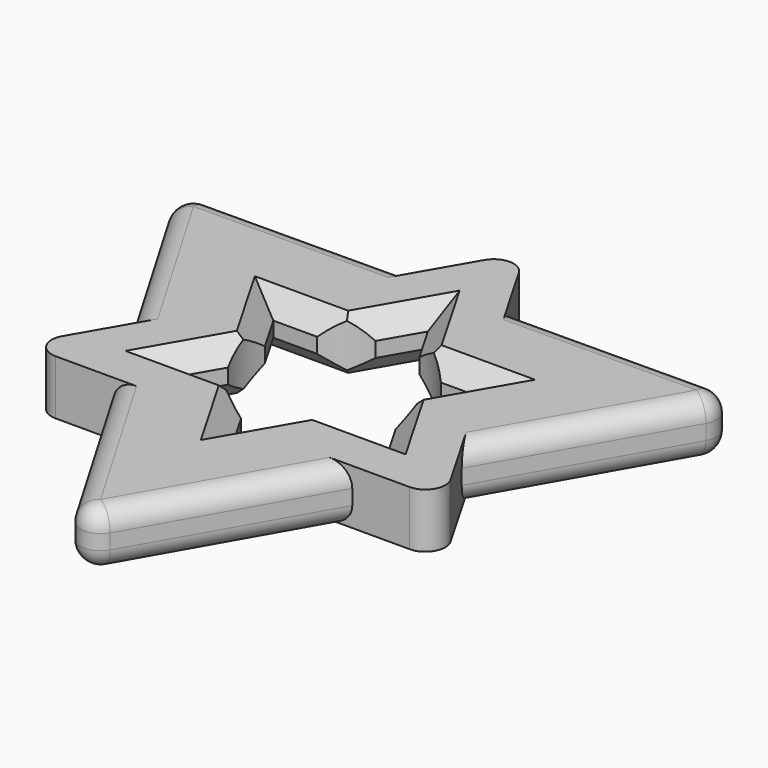
from build123d import *

# Parameters (mm, degrees)
F1_DEPTH      = 7
F2_T4_DEPTH   = 18.6684863764
F2_T9_DEPTH   = 18.6684863764
F2_T14_DEPTH  = 18.6684863764
F2_T19_DEPTH  = 18.6684863764
F2_T24_DEPTH  = 18.6684863764
F2_T29_DEPTH  = 18.6684863764
F2_T34_DEPTH  = 18.6684863764
F2_T39_DEPTH  = 18.6684863764
F2_T44_DEPTH  = 18.6684863764
F2_T49_DEPTH  = 18.6684863764
F2_T54_DEPTH  = 18.6684863764
F2_T59_DEPTH  = 18.6684863764
F2_T64_DEPTH  = 18.6684863764
F2_T69_DEPTH  = 18.6684863764
F2_T74_DEPTH  = 18.6684863764
F2_T79_DEPTH  = 18.6684863764
F2_T84_DEPTH  = 18.6684863764
F2_T89_DEPTH  = 18.6684863764
F2_T94_DEPTH  = 18.6684863764
F2_T99_DEPTH  = 18.6684863764
F2_T104_DEPTH = 18.6684863764
F2_T109_DEPTH = 18.6684863764
F2_T114_DEPTH = 18.6684863764
F2_T119_DEPTH = 18.6684863764
F2_T125_DEPTH = 18.6684863764
F2_T129_DEPTH = 18.6684863764
F2_T136_DEPTH = 18.6684863764
F2_T140_DEPTH = 18.6684863764
F2_T147_DEPTH = 18.6684863764
F2_T151_DEPTH = 18.6684863764
F2_T158_DEPTH = 18.6684863764
F2_T162_DEPTH = 18.6684863764
F2_T169_DEPTH = 18.6684863764
F2_T173_DEPTH = 18.6684863764
F2_T180_DEPTH = 18.6684863764
F2_T184_DEPTH = 18.6684863764
F2_T191_DEPTH = 18.6684863764
F2_T195_DEPTH = 18.6684863764
F2_T202_DEPTH = 18.6684863764
F2_T206_DEPTH = 18.6684863764
F2_T213_DEPTH = 18.6684863764
F2_T217_DEPTH = 18.6684863764
F2_T224_DEPTH = 18.6684863764
F2_T228_DEPTH = 18.6684863764
F2_T235_DEPTH = 18.6684863764
F2_T239_DEPTH = 18.6684863764
F2_T246_DEPTH = 18.6684863764
F2_T250_DEPTH = 18.6684863764
F3_R          = 2.54
F4_T1_DEPTH   = 28.9970452561
F4_T3_DEPTH   = 1.92
F4_T8_DEPTH   = 2.54
F4_T14_DEPTH  = 2.54
F4_T20_DEPTH  = 2.54
F4_T26_DEPTH  = 2.54
F4_T32_DEPTH  = 2.54
F4_T38_DEPTH  = 2.54


# Not quite as in the source:
# - a fillet or chamfer that OpenCascade refuses, or shapes differently, is made with other operations: its cross-section is extruded or revolved along the edge and cut away or added
# - two fillets or chamfers of one size are made in one step


with BuildPart() as f1:
    # F0 (on Top) → F1 (new body)
    with BuildSketch(Plane.XY):
        with BuildLine():
            Line((21.1293552338, -5.3833303027), (13.5159660258, 7.8034466234))
            ThreePointArc((13.5159660258, 7.8034466234), (15.0751012551, 4.0393612071), (15.6068932467, 0))
            ThreePointArc((15.6068932467, 0), (15.0751012551, -4.0393612071), (13.5159660258, -7.8034466234))
            ThreePointArc((13.5159660258, -7.8034466234), (7.8034466234, -13.5159660258), (0, -15.6068932467))
            Line((0, -15.6068932467), (15.3081617463, -15.6068932467))
            Line((15.3081617463, -15.6068932467), (21.1293552338, -5.3833303027))
        make_face()
        with BuildLine():
            ThreePointArc((0, 15.6068932467), (7.8034466234, 13.5159660258), (13.5159660258, 7.8034466234))
            Line((13.5159660258, 7.8034466234), (5.8618851526, 21.0607035809))
            Line((5.8618851526, 21.0607035809), (-5.9025768178, 20.9902235494))
            Line((-5.9025768178, 20.9902235494), (-13.5159660258, 7.8034466234))
            ThreePointArc((-13.5159660258, 7.8034466234), (-7.8034466234, 13.5159660258), (0, 15.6068932467))
        make_face()
        Polygon((5.8618851526, 21.0607035809), (13.5159660258, 7.8034466234), (21.1293552338, -5.3833303027), (36.2901170268, 21.2429968933), align=None)
        Polygon((-5.9025768178, 20.9902235494), (5.8618851526, 21.0607035809), (0, 31.2137864934), align=None)
        Polygon((27.0319320516, -15.6068932467), (21.1293552338, -5.3833303027), (15.3081617463, -15.6068932467), align=None)
        with BuildLine():
            Line((-15.226778416, -15.6068932467), (0, -15.6068932467))
            ThreePointArc((0, -15.6068932467), (-7.8034466234, -13.5159660258), (-13.5159660258, -7.8034466234))
            ThreePointArc((-13.5159660258, -7.8034466234), (-15.6068932467, 0), (-13.5159660258, 7.8034466234))
            Line((-13.5159660258, 7.8034466234), (-21.170046899, -5.4538103342))
            Line((-21.170046899, -5.4538103342), (-15.226778416, -15.6068932467))
        make_face()
        Polygon((15.3081617463, -15.6068932467), (0, -15.6068932467), (-15.226778416, -15.6068932467), (0.2519164487, -42.0496616981), align=None)
        Polygon((-21.170046899, -5.4538103342), (-13.5159660258, 7.8034466234), (-5.9025768178, 20.9902235494), (-36.5420334755, 20.8066648049), align=None)
        Polygon((-27.0319320516, -15.6068932467), (-15.226778416, -15.6068932467), (-21.170046899, -5.4538103342), align=None)
        with BuildLine():
            Line((-10.7137976271, 2.9499485854), (-13.5159660258, 7.8034466234))
            ThreePointArc((-13.5159660258, 7.8034466234), (-15.6068932467, 0), (-13.5159660258, -7.8034466234))
            Line((-13.5159660258, -7.8034466234), (-10.7137976271, -2.9499485854))
            ThreePointArc((-10.7137976271, -2.9499485854), (-11.1125, 0), (-10.7137976271, 2.9499485854))
        make_face()
        with BuildLine():
            ThreePointArc((2.8021683987, 10.7533952087), (5.55625, 9.6237072996), (7.9116292283, 7.8034466234))
            Line((7.9116292283, 7.8034466234), (13.5159660258, 7.8034466234))
            ThreePointArc((13.5159660258, 7.8034466234), (7.8034466234, 13.5159660258), (0, 15.6068932467))
            Line((0, 15.6068932467), (2.8021683987, 10.7533952087))
        make_face()
        with BuildLine():
            Line((13.5159660258, -7.8034466234), (7.9116292283, -7.8034466234))
            ThreePointArc((7.9116292283, -7.8034466234), (5.55625, -9.6237072996), (2.8021683987, -10.7533952087))
            Line((2.8021683987, -10.7533952087), (0, -15.6068932467))
            ThreePointArc((0, -15.6068932467), (7.8034466234, -13.5159660258), (13.5159660258, -7.8034466234))
        make_face()
        with BuildLine():
            ThreePointArc((-13.5159660258, -7.8034466234), (-7.8034466234, -13.5159660258), (0, -15.6068932467))
            Line((0, -15.6068932467), (-2.8021683987, -10.7533952087))
            ThreePointArc((-2.8021683987, -10.7533952087), (-5.55625, -9.6237072996), (-7.9116292283, -7.8034466234))
            Line((-7.9116292283, -7.8034466234), (-13.5159660258, -7.8034466234))
        make_face()
        with BuildLine():
            ThreePointArc((10.7137976271, 2.9499485854), (11.0123733223, 1.4883850509), (11.1125, 0))
            ThreePointArc((11.1125, 0), (11.0123733223, -1.4883850509), (10.7137976271, -2.9499485854))
            Line((10.7137976271, -2.9499485854), (13.5159660258, -7.8034466234))
            ThreePointArc((13.5159660258, -7.8034466234), (15.0751012551, -4.0393612071), (15.6068932467, 0))
            ThreePointArc((15.6068932467, 0), (15.0751012551, 4.0393612071), (13.5159660258, 7.8034466234))
            Line((13.5159660258, 7.8034466234), (10.7137976271, 2.9499485854))
        make_face()
        with BuildLine():
            Line((-2.8021683987, 10.7533952087), (0, 15.6068932467))
            ThreePointArc((0, 15.6068932467), (-7.8034466234, 13.5159660258), (-13.5159660258, 7.8034466234))
            Line((-13.5159660258, 7.8034466234), (-7.9116292283, 7.8034466234))
            ThreePointArc((-7.9116292283, 7.8034466234), (-5.55625, 9.6237072996), (-2.8021683987, 10.7533952087))
        make_face()
    extrude(amount=F1_DEPTH)

    # F2: chamfer of 2.54 on 24 edges, made by hand


with BuildPart() as f2_tool2:
    # F2_s3 → F2_t4 (new body)
    with BuildSketch(Plane.YZ.offset(-20.0480408152)):
        Polygon((7.8034466234, 4.46), (10.3434466234, 7), (7.8034466234, 7), align=None)
    extrude(amount=F2_T4_DEPTH)

    split(bisect_by=Plane(origin=(-6.7579830129, -3.9017233117, 0), x_dir=(0, 0, 1), z_dir=(0.8660254038, 0.5, 0)), keep=Keep.TOP)


with BuildPart() as f1_1:
    add(f1.part)

    # F2_t1: cut F2_tool2
    add(f2_tool2.part, mode=Mode.SUBTRACT)


with BuildPart() as f2_tool7:
    # F2_s8 → F2_t9 (new body)
    with BuildSketch(Plane.YZ.offset(-20.0480408152)):
        Polygon((7.8034466234, 2.54), (10.3434466234, 0), (7.8034466234, 0), align=None)
    extrude(amount=F2_T9_DEPTH)

    split(bisect_by=Plane(origin=(-6.7579830129, -3.9017233117, 0), x_dir=(0, 0, 1), z_dir=(0.8660254038, 0.5, 0)), keep=Keep.TOP)


with BuildPart() as f1_2:
    add(f1_1.part)

    # F2_t6: cut F2_tool7
    add(f2_tool7.part, mode=Mode.SUBTRACT)


with BuildPart() as f2_tool12:
    # F2_s13 → F2_t14 (new body)
    with BuildSketch(Plane(origin=(-0.6897772194, 1.19472919, 0), x_dir=(0, 0, 1), z_dir=(-0.5, 0.8660254038, 0))):
        Polygon((2.54, -7.8034466234), (0, -10.3434466234), (0, -7.8034466234), align=None)
    extrude(amount=F2_T14_DEPTH)

    split(bisect_by=Plane.XZ.offset(-7.8034466234), keep=Keep.TOP)


with BuildPart() as f1_3:
    add(f1_2.part)

    # F2_t11: cut F2_tool12
    add(f2_tool12.part, mode=Mode.SUBTRACT)


with BuildPart() as f2_tool17:
    # F2_s18 → F2_t19 (new body)
    with BuildSketch(Plane.YZ.offset(-1.3795544389)):
        Polygon((-7.8034466234, 2.54), (-10.3434466234, 0), (-7.8034466234, 0), align=None)
    extrude(amount=-F2_T19_DEPTH)

    split(bisect_by=Plane(origin=(-6.7579830129, 3.9017233117, 0), x_dir=(0, 0, 1), z_dir=(0.8660254038, -0.5, 0)), keep=Keep.TOP)


with BuildPart() as f1_4:
    add(f1_3.part)

    # F2_t16: cut F2_tool17
    add(f2_tool17.part, mode=Mode.SUBTRACT)


with BuildPart() as f2_tool22:
    # F2_s23 → F2_t24 (new body)
    with BuildSketch(Plane(origin=(-10.0240204076, -17.3621126421, 0), x_dir=(0, 0, 1), z_dir=(0.5, 0.8660254038, 0))):
        Polygon((2.54, -7.8034466234), (0, -10.3434466234), (0, -7.8034466234), align=None)
    extrude(amount=F2_T24_DEPTH)

    split(bisect_by=Plane.XZ.offset(7.8034466234), keep=Keep.BOTTOM)


with BuildPart() as f1_5:
    add(f1_4.part)

    # F2_t21: cut F2_tool22
    add(f2_tool22.part, mode=Mode.SUBTRACT)


with BuildPart() as f2_tool27:
    # F2_s28 → F2_t29 (new body)
    with BuildSketch(Plane(origin=(10.0240204076, -17.3621126421, 0), x_dir=(0, 0, 1), z_dir=(-0.5, 0.8660254038, 0))):
        Polygon((2.54, -7.8034466234), (0, -10.3434466234), (0, -7.8034466234), align=None)
    extrude(amount=F2_T29_DEPTH)

    split(bisect_by=Plane(origin=(6.7579830129, -3.9017233117, 0), x_dir=(0, 0, 1), z_dir=(-0.8660254038, 0.5, 0)), keep=Keep.TOP)


with BuildPart() as f1_6:
    add(f1_5.part)

    # F2_t26: cut F2_tool27
    add(f2_tool27.part, mode=Mode.SUBTRACT)


with BuildPart() as f2_tool32:
    # F2_s33 → F2_t34 (new body)
    with BuildSketch(Plane(origin=(-0.6897772194, -1.19472919, 0), x_dir=(0, 0, 1), z_dir=(-0.5, -0.8660254038, 0))):
        Polygon((2.54, -7.8034466234), (0, -10.3434466234), (0, -7.8034466234), align=None)
    extrude(amount=F2_T34_DEPTH)

    split(bisect_by=Plane(origin=(-6.7579830129, -3.9017233117, 0), x_dir=(0, 0, 1), z_dir=(0.8660254038, 0.5, 0)), keep=Keep.TOP)


with BuildPart() as f1_7:
    add(f1_6.part)

    # F2_t31: cut F2_tool32
    add(f2_tool32.part, mode=Mode.SUBTRACT)


with BuildPart() as f2_tool37:
    # F2_s38 → F2_t39 (new body)
    with BuildSketch(Plane.YZ.offset(20.0480408152)):
        Polygon((-7.8034466234, 2.54), (-10.3434466234, 0), (-7.8034466234, 0), align=None)
    extrude(amount=-F2_T39_DEPTH)

    split(bisect_by=Plane(origin=(6.7579830129, 3.9017233117, 0), x_dir=(0, 0, 1), z_dir=(-0.8660254038, -0.5, 0)), keep=Keep.TOP)


with BuildPart() as f1_8:
    add(f1_7.part)

    # F2_t36: cut F2_tool37
    add(f2_tool37.part, mode=Mode.SUBTRACT)


with BuildPart() as f2_tool42:
    # F2_s43 → F2_t44 (new body)
    with BuildSketch(Plane(origin=(0.6897772194, -1.19472919, 0), x_dir=(0, 0, 1), z_dir=(0.5, -0.8660254038, 0))):
        Polygon((2.54, -7.8034466234), (0, -10.3434466234), (0, -7.8034466234), align=None)
    extrude(amount=F2_T44_DEPTH)

    split(bisect_by=Plane.XZ.offset(7.8034466234), keep=Keep.BOTTOM)


with BuildPart() as f1_9:
    add(f1_8.part)

    # F2_t41: cut F2_tool42
    add(f2_tool42.part, mode=Mode.SUBTRACT)


with BuildPart() as f2_tool47:
    # F2_s48 → F2_t49 (new body)
    with BuildSketch(Plane(origin=(10.0240204076, 17.3621126421, 0), x_dir=(0, 0, 1), z_dir=(-0.5, -0.8660254038, 0))):
        Polygon((2.54, -7.8034466234), (0, -10.3434466234), (0, -7.8034466234), align=None)
    extrude(amount=F2_T49_DEPTH)

    split(bisect_by=Plane.XZ.offset(-7.8034466234), keep=Keep.TOP)


with BuildPart() as f1_10:
    add(f1_9.part)

    # F2_t46: cut F2_tool47
    add(f2_tool47.part, mode=Mode.SUBTRACT)


with BuildPart() as f2_tool52:
    # F2_s53 → F2_t54 (new body)
    with BuildSketch(Plane.YZ.offset(1.3795544389)):
        Polygon((7.8034466234, 2.54), (10.3434466234, 0), (7.8034466234, 0), align=None)
    extrude(amount=F2_T54_DEPTH)

    split(bisect_by=Plane(origin=(6.7579830129, -3.9017233117, 0), x_dir=(0, 0, 1), z_dir=(-0.8660254038, 0.5, 0)), keep=Keep.TOP)


with BuildPart() as f1_11:
    add(f1_10.part)

    # F2_t51: cut F2_tool52
    add(f2_tool52.part, mode=Mode.SUBTRACT)


with BuildPart() as f2_tool57:
    # F2_s58 → F2_t59 (new body)
    with BuildSketch(Plane(origin=(-10.0240204076, 17.3621126421, 0), x_dir=(0, 0, 1), z_dir=(0.5, -0.8660254038, 0))):
        Polygon((2.54, -7.8034466234), (0, -10.3434466234), (0, -7.8034466234), align=None)
    extrude(amount=F2_T59_DEPTH)

    split(bisect_by=Plane(origin=(-6.7579830129, 3.9017233117, 0), x_dir=(0, 0, 1), z_dir=(0.8660254038, -0.5, 0)), keep=Keep.TOP)


with BuildPart() as f1_12:
    add(f1_11.part)

    # F2_t56: cut F2_tool57
    add(f2_tool57.part, mode=Mode.SUBTRACT)


with BuildPart() as f2_tool62:
    # F2_s63 → F2_t64 (new body)
    with BuildSketch(Plane(origin=(0.6897772194, 1.19472919, 0), x_dir=(0, 0, 1), z_dir=(0.5, 0.8660254038, 0))):
        Polygon((2.54, -7.8034466234), (0, -10.3434466234), (0, -7.8034466234), align=None)
    extrude(amount=F2_T64_DEPTH)

    split(bisect_by=Plane(origin=(6.7579830129, 3.9017233117, 0), x_dir=(0, 0, 1), z_dir=(-0.8660254038, -0.5, 0)), keep=Keep.TOP)


with BuildPart() as f1_13:
    add(f1_12.part)

    # F2_t61: cut F2_tool62
    add(f2_tool62.part, mode=Mode.SUBTRACT)


with BuildPart() as f2_tool67:
    # F2_s68 → F2_t69 (new body)
    with BuildSketch(Plane(origin=(0.6897772194, 1.19472919, 0), x_dir=(0, 0, 1), z_dir=(0.5, 0.8660254038, 0))):
        Polygon((4.46, -7.8034466234), (7, -10.3434466234), (7, -7.8034466234), align=None)
    extrude(amount=F2_T69_DEPTH)

    split(bisect_by=Plane(origin=(6.7579830129, 3.9017233117, 0), x_dir=(0, 0, 1), z_dir=(-0.8660254038, -0.5, 0)), keep=Keep.TOP)


with BuildPart() as f1_14:
    add(f1_13.part)

    # F2_t66: cut F2_tool67
    add(f2_tool67.part, mode=Mode.SUBTRACT)


with BuildPart() as f2_tool72:
    # F2_s73 → F2_t74 (new body)
    with BuildSketch(Plane(origin=(-10.0240204076, 17.3621126421, 0), x_dir=(0, 0, 1), z_dir=(0.5, -0.8660254038, 0))):
        Polygon((4.46, -7.8034466234), (7, -10.3434466234), (7, -7.8034466234), align=None)
    extrude(amount=F2_T74_DEPTH)

    split(bisect_by=Plane(origin=(-6.7579830129, 3.9017233117, 0), x_dir=(0, 0, 1), z_dir=(0.8660254038, -0.5, 0)), keep=Keep.TOP)


with BuildPart() as f1_15:
    add(f1_14.part)

    # F2_t71: cut F2_tool72
    add(f2_tool72.part, mode=Mode.SUBTRACT)


with BuildPart() as f2_tool77:
    # F2_s78 → F2_t79 (new body)
    with BuildSketch(Plane.YZ.offset(1.3795544389)):
        Polygon((7.8034466234, 4.46), (10.3434466234, 7), (7.8034466234, 7), align=None)
    extrude(amount=F2_T79_DEPTH)

    split(bisect_by=Plane(origin=(6.7579830129, -3.9017233117, 0), x_dir=(0, 0, 1), z_dir=(-0.8660254038, 0.5, 0)), keep=Keep.TOP)


with BuildPart() as f1_16:
    add(f1_15.part)

    # F2_t76: cut F2_tool77
    add(f2_tool77.part, mode=Mode.SUBTRACT)


with BuildPart() as f2_tool82:
    # F2_s83 → F2_t84 (new body)
    with BuildSketch(Plane(origin=(10.0240204076, 17.3621126421, 0), x_dir=(0, 0, 1), z_dir=(-0.5, -0.8660254038, 0))):
        Polygon((4.46, -7.8034466234), (7, -10.3434466234), (7, -7.8034466234), align=None)
    extrude(amount=F2_T84_DEPTH)

    split(bisect_by=Plane.XZ.offset(-7.8034466234), keep=Keep.TOP)


with BuildPart() as f1_17:
    add(f1_16.part)

    # F2_t81: cut F2_tool82
    add(f2_tool82.part, mode=Mode.SUBTRACT)


with BuildPart() as f2_tool87:
    # F2_s88 → F2_t89 (new body)
    with BuildSketch(Plane(origin=(0.6897772194, -1.19472919, 0), x_dir=(0, 0, 1), z_dir=(0.5, -0.8660254038, 0))):
        Polygon((4.46, -7.8034466234), (7, -10.3434466234), (7, -7.8034466234), align=None)
    extrude(amount=F2_T89_DEPTH)

    split(bisect_by=Plane.XZ.offset(7.8034466234), keep=Keep.BOTTOM)


with BuildPart() as f1_18:
    add(f1_17.part)

    # F2_t86: cut F2_tool87
    add(f2_tool87.part, mode=Mode.SUBTRACT)


with BuildPart() as f2_tool92:
    # F2_s93 → F2_t94 (new body)
    with BuildSketch(Plane.YZ.offset(20.0480408152)):
        Polygon((-7.8034466234, 4.46), (-10.3434466234, 7), (-7.8034466234, 7), align=None)
    extrude(amount=-F2_T94_DEPTH)

    split(bisect_by=Plane(origin=(6.7579830129, 3.9017233117, 0), x_dir=(0, 0, 1), z_dir=(-0.8660254038, -0.5, 0)), keep=Keep.TOP)


with BuildPart() as f1_19:
    add(f1_18.part)

    # F2_t91: cut F2_tool92
    add(f2_tool92.part, mode=Mode.SUBTRACT)


with BuildPart() as f2_tool97:
    # F2_s98 → F2_t99 (new body)
    with BuildSketch(Plane(origin=(-0.6897772194, -1.19472919, 0), x_dir=(0, 0, 1), z_dir=(-0.5, -0.8660254038, 0))):
        Polygon((4.46, -7.8034466234), (7, -10.3434466234), (7, -7.8034466234), align=None)
    extrude(amount=F2_T99_DEPTH)

    split(bisect_by=Plane(origin=(-6.7579830129, -3.9017233117, 0), x_dir=(0, 0, 1), z_dir=(0.8660254038, 0.5, 0)), keep=Keep.TOP)


with BuildPart() as f1_20:
    add(f1_19.part)

    # F2_t96: cut F2_tool97
    add(f2_tool97.part, mode=Mode.SUBTRACT)


with BuildPart() as f2_tool102:
    # F2_s103 → F2_t104 (new body)
    with BuildSketch(Plane(origin=(10.0240204076, -17.3621126421, 0), x_dir=(0, 0, 1), z_dir=(-0.5, 0.8660254038, 0))):
        Polygon((4.46, -7.8034466234), (7, -10.3434466234), (7, -7.8034466234), align=None)
    extrude(amount=F2_T104_DEPTH)

    split(bisect_by=Plane(origin=(6.7579830129, -3.9017233117, 0), x_dir=(0, 0, 1), z_dir=(-0.8660254038, 0.5, 0)), keep=Keep.TOP)


with BuildPart() as f1_21:
    add(f1_20.part)

    # F2_t101: cut F2_tool102
    add(f2_tool102.part, mode=Mode.SUBTRACT)


with BuildPart() as f2_tool107:
    # F2_s108 → F2_t109 (new body)
    with BuildSketch(Plane.YZ.offset(-1.3795544389)):
        Polygon((-7.8034466234, 4.46), (-10.3434466234, 7), (-7.8034466234, 7), align=None)
    extrude(amount=-F2_T109_DEPTH)

    split(bisect_by=Plane(origin=(-6.7579830129, 3.9017233117, 0), x_dir=(0, 0, 1), z_dir=(0.8660254038, -0.5, 0)), keep=Keep.TOP)


with BuildPart() as f1_22:
    add(f1_21.part)

    # F2_t106: cut F2_tool107
    add(f2_tool107.part, mode=Mode.SUBTRACT)


with BuildPart() as f2_tool112:
    # F2_s113 → F2_t114 (new body)
    with BuildSketch(Plane(origin=(-10.0240204076, -17.3621126421, 0), x_dir=(0, 0, 1), z_dir=(0.5, 0.8660254038, 0))):
        Polygon((4.46, -7.8034466234), (7, -10.3434466234), (7, -7.8034466234), align=None)
    extrude(amount=F2_T114_DEPTH)

    split(bisect_by=Plane.XZ.offset(7.8034466234), keep=Keep.BOTTOM)


with BuildPart() as f1_23:
    add(f1_22.part)

    # F2_t111: cut F2_tool112
    add(f2_tool112.part, mode=Mode.SUBTRACT)


with BuildPart() as f2_tool117:
    # F2_s118 → F2_t119 (new body)
    with BuildSketch(Plane(origin=(-0.6897772194, 1.19472919, 0), x_dir=(0, 0, 1), z_dir=(-0.5, 0.8660254038, 0))):
        Polygon((4.46, -7.8034466234), (7, -10.3434466234), (7, -7.8034466234), align=None)
    extrude(amount=F2_T119_DEPTH)

    split(bisect_by=Plane.XZ.offset(-7.8034466234), keep=Keep.TOP)


with BuildPart() as f1_24:
    add(f1_23.part)

    # F2_t116: cut F2_tool117
    add(f2_tool117.part, mode=Mode.SUBTRACT)


with BuildPart() as f2_tool123:
    # F2_s124 → F2_t125 (new body)
    with BuildSketch(Plane(origin=(-0.6897772194, 1.19472919, 0), x_dir=(0, 0, 1), z_dir=(-0.5, 0.8660254038, 0))):
        Polygon((4.46, -7.8034466234), (7, -10.3434466234), (7, -7.8034466234), align=None)
    extrude(amount=F2_T125_DEPTH)

    split(bisect_by=Plane.XZ.offset(-7.8034466234), keep=Keep.BOTTOM)


with BuildPart() as f2_tool127:
    # F2_s128 → F2_t129 (new body)
    with BuildSketch(Plane.YZ.offset(-20.0480408152)):
        Polygon((7.8034466234, 4.46), (10.3434466234, 7), (7.8034466234, 7), align=None)
    extrude(amount=F2_T129_DEPTH)

    split(bisect_by=Plane(origin=(-6.7579830129, -3.9017233117, 0), x_dir=(0, 0, 1), z_dir=(-0.8660254038, -0.5, 0)), keep=Keep.TOP)


with BuildPart() as f2_tool123_1:
    add(f2_tool123.part)

    # F2_t131: intersect F2_tool127
    add(f2_tool127.part, mode=Mode.INTERSECT)


with BuildPart() as f1_25:
    add(f1_24.part)

    # F2_t121: cut F2_tool123
    add(f2_tool123_1.part, mode=Mode.SUBTRACT)


with BuildPart() as f2_tool134:
    # F2_s135 → F2_t136 (new body)
    with BuildSketch(Plane(origin=(-0.6897772194, 1.19472919, 0), x_dir=(0, 0, 1), z_dir=(-0.5, 0.8660254038, 0))):
        Polygon((2.54, -7.8034466234), (0, -10.3434466234), (0, -7.8034466234), align=None)
    extrude(amount=F2_T136_DEPTH)

    split(bisect_by=Plane.XZ.offset(-7.8034466234), keep=Keep.BOTTOM)


with BuildPart() as f2_tool138:
    # F2_s139 → F2_t140 (new body)
    with BuildSketch(Plane.YZ.offset(-20.0480408152)):
        Polygon((7.8034466234, 2.54), (10.3434466234, 0), (7.8034466234, 0), align=None)
    extrude(amount=F2_T140_DEPTH)

    split(bisect_by=Plane(origin=(-6.7579830129, -3.9017233117, 0), x_dir=(0, 0, 1), z_dir=(-0.8660254038, -0.5, 0)), keep=Keep.TOP)


with BuildPart() as f2_tool134_1:
    add(f2_tool134.part)

    # F2_t142: intersect F2_tool138
    add(f2_tool138.part, mode=Mode.INTERSECT)


with BuildPart() as f1_26:
    add(f1_25.part)

    # F2_t132: cut F2_tool134
    add(f2_tool134_1.part, mode=Mode.SUBTRACT)


with BuildPart() as f2_tool145:
    # F2_s146 → F2_t147 (new body)
    with BuildSketch(Plane.YZ.offset(-1.3795544389)):
        Polygon((-7.8034466234, 2.54), (-10.3434466234, 0), (-7.8034466234, 0), align=None)
    extrude(amount=-F2_T147_DEPTH)

    split(bisect_by=Plane(origin=(-6.7579830129, 3.9017233117, 0), x_dir=(0, 0, 1), z_dir=(-0.8660254038, 0.5, 0)), keep=Keep.TOP)


with BuildPart() as f2_tool149:
    # F2_s150 → F2_t151 (new body)
    with BuildSketch(Plane(origin=(-10.0240204076, -17.3621126421, 0), x_dir=(0, 0, 1), z_dir=(0.5, 0.8660254038, 0))):
        Polygon((2.54, -7.8034466234), (0, -10.3434466234), (0, -7.8034466234), align=None)
    extrude(amount=F2_T151_DEPTH)

    split(bisect_by=Plane.XZ.offset(7.8034466234), keep=Keep.TOP)


with BuildPart() as f2_tool145_1:
    add(f2_tool145.part)

    # F2_t153: intersect F2_tool149
    add(f2_tool149.part, mode=Mode.INTERSECT)


with BuildPart() as f1_27:
    add(f1_26.part)

    # F2_t143: cut F2_tool145
    add(f2_tool145_1.part, mode=Mode.SUBTRACT)


with BuildPart() as f2_tool156:
    # F2_s157 → F2_t158 (new body)
    with BuildSketch(Plane(origin=(-0.6897772194, -1.19472919, 0), x_dir=(0, 0, 1), z_dir=(-0.5, -0.8660254038, 0))):
        Polygon((2.54, -7.8034466234), (0, -10.3434466234), (0, -7.8034466234), align=None)
    extrude(amount=F2_T158_DEPTH)

    split(bisect_by=Plane(origin=(-6.7579830129, -3.9017233117, 0), x_dir=(0, 0, 1), z_dir=(-0.8660254038, -0.5, 0)), keep=Keep.TOP)


with BuildPart() as f2_tool160:
    # F2_s161 → F2_t162 (new body)
    with BuildSketch(Plane(origin=(10.0240204076, -17.3621126421, 0), x_dir=(0, 0, 1), z_dir=(-0.5, 0.8660254038, 0))):
        Polygon((2.54, -7.8034466234), (0, -10.3434466234), (0, -7.8034466234), align=None)
    extrude(amount=F2_T162_DEPTH)

    split(bisect_by=Plane(origin=(6.7579830129, -3.9017233117, 0), x_dir=(0, 0, 1), z_dir=(0.8660254038, -0.5, 0)), keep=Keep.TOP)


with BuildPart() as f2_tool156_1:
    add(f2_tool156.part)

    # F2_t164: intersect F2_tool160
    add(f2_tool160.part, mode=Mode.INTERSECT)


with BuildPart() as f1_28:
    add(f1_27.part)

    # F2_t154: cut F2_tool156
    add(f2_tool156_1.part, mode=Mode.SUBTRACT)


with BuildPart() as f2_tool167:
    # F2_s168 → F2_t169 (new body)
    with BuildSketch(Plane(origin=(0.6897772194, -1.19472919, 0), x_dir=(0, 0, 1), z_dir=(0.5, -0.8660254038, 0))):
        Polygon((2.54, -7.8034466234), (0, -10.3434466234), (0, -7.8034466234), align=None)
    extrude(amount=F2_T169_DEPTH)

    split(bisect_by=Plane.XZ.offset(7.8034466234), keep=Keep.TOP)


with BuildPart() as f2_tool171:
    # F2_s172 → F2_t173 (new body)
    with BuildSketch(Plane.YZ.offset(20.0480408152)):
        Polygon((-7.8034466234, 2.54), (-10.3434466234, 0), (-7.8034466234, 0), align=None)
    extrude(amount=-F2_T173_DEPTH)

    split(bisect_by=Plane(origin=(6.7579830129, 3.9017233117, 0), x_dir=(0, 0, 1), z_dir=(0.8660254038, 0.5, 0)), keep=Keep.TOP)


with BuildPart() as f2_tool167_1:
    add(f2_tool167.part)

    # F2_t175: intersect F2_tool171
    add(f2_tool171.part, mode=Mode.INTERSECT)


with BuildPart() as f1_29:
    add(f1_28.part)

    # F2_t165: cut F2_tool167
    add(f2_tool167_1.part, mode=Mode.SUBTRACT)


with BuildPart() as f2_tool178:
    # F2_s179 → F2_t180 (new body)
    with BuildSketch(Plane.YZ.offset(1.3795544389)):
        Polygon((7.8034466234, 2.54), (10.3434466234, 0), (7.8034466234, 0), align=None)
    extrude(amount=F2_T180_DEPTH)

    split(bisect_by=Plane(origin=(6.7579830129, -3.9017233117, 0), x_dir=(0, 0, 1), z_dir=(0.8660254038, -0.5, 0)), keep=Keep.TOP)


with BuildPart() as f2_tool182:
    # F2_s183 → F2_t184 (new body)
    with BuildSketch(Plane(origin=(10.0240204076, 17.3621126421, 0), x_dir=(0, 0, 1), z_dir=(-0.5, -0.8660254038, 0))):
        Polygon((2.54, -7.8034466234), (0, -10.3434466234), (0, -7.8034466234), align=None)
    extrude(amount=F2_T184_DEPTH)

    split(bisect_by=Plane.XZ.offset(-7.8034466234), keep=Keep.BOTTOM)


with BuildPart() as f2_tool178_1:
    add(f2_tool178.part)

    # F2_t186: intersect F2_tool182
    add(f2_tool182.part, mode=Mode.INTERSECT)


with BuildPart() as f1_30:
    add(f1_29.part)

    # F2_t176: cut F2_tool178
    add(f2_tool178_1.part, mode=Mode.SUBTRACT)


with BuildPart() as f2_tool189:
    # F2_s190 → F2_t191 (new body)
    with BuildSketch(Plane(origin=(-10.0240204076, 17.3621126421, 0), x_dir=(0, 0, 1), z_dir=(0.5, -0.8660254038, 0))):
        Polygon((2.54, -7.8034466234), (0, -10.3434466234), (0, -7.8034466234), align=None)
    extrude(amount=F2_T191_DEPTH)

    split(bisect_by=Plane(origin=(-6.7579830129, 3.9017233117, 0), x_dir=(0, 0, 1), z_dir=(-0.8660254038, 0.5, 0)), keep=Keep.TOP)


with BuildPart() as f2_tool193:
    # F2_s194 → F2_t195 (new body)
    with BuildSketch(Plane(origin=(0.6897772194, 1.19472919, 0), x_dir=(0, 0, 1), z_dir=(0.5, 0.8660254038, 0))):
        Polygon((2.54, -7.8034466234), (0, -10.3434466234), (0, -7.8034466234), align=None)
    extrude(amount=F2_T195_DEPTH)

    split(bisect_by=Plane(origin=(6.7579830129, 3.9017233117, 0), x_dir=(0, 0, 1), z_dir=(0.8660254038, 0.5, 0)), keep=Keep.TOP)


with BuildPart() as f2_tool189_1:
    add(f2_tool189.part)

    # F2_t197: intersect F2_tool193
    add(f2_tool193.part, mode=Mode.INTERSECT)


with BuildPart() as f1_31:
    add(f1_30.part)

    # F2_t187: cut F2_tool189
    add(f2_tool189_1.part, mode=Mode.SUBTRACT)


with BuildPart() as f2_tool200:
    # F2_s201 → F2_t202 (new body)
    with BuildSketch(Plane(origin=(-10.0240204076, 17.3621126421, 0), x_dir=(0, 0, 1), z_dir=(0.5, -0.8660254038, 0))):
        Polygon((4.46, -7.8034466234), (7, -10.3434466234), (7, -7.8034466234), align=None)
    extrude(amount=F2_T202_DEPTH)

    split(bisect_by=Plane(origin=(-6.7579830129, 3.9017233117, 0), x_dir=(0, 0, 1), z_dir=(-0.8660254038, 0.5, 0)), keep=Keep.TOP)


with BuildPart() as f2_tool204:
    # F2_s205 → F2_t206 (new body)
    with BuildSketch(Plane(origin=(0.6897772194, 1.19472919, 0), x_dir=(0, 0, 1), z_dir=(0.5, 0.8660254038, 0))):
        Polygon((4.46, -7.8034466234), (7, -10.3434466234), (7, -7.8034466234), align=None)
    extrude(amount=F2_T206_DEPTH)

    split(bisect_by=Plane(origin=(6.7579830129, 3.9017233117, 0), x_dir=(0, 0, 1), z_dir=(0.8660254038, 0.5, 0)), keep=Keep.TOP)


with BuildPart() as f2_tool200_1:
    add(f2_tool200.part)

    # F2_t208: intersect F2_tool204
    add(f2_tool204.part, mode=Mode.INTERSECT)


with BuildPart() as f1_32:
    add(f1_31.part)

    # F2_t198: cut F2_tool200
    add(f2_tool200_1.part, mode=Mode.SUBTRACT)


with BuildPart() as f2_tool211:
    # F2_s212 → F2_t213 (new body)
    with BuildSketch(Plane.YZ.offset(1.3795544389)):
        Polygon((7.8034466234, 4.46), (10.3434466234, 7), (7.8034466234, 7), align=None)
    extrude(amount=F2_T213_DEPTH)

    split(bisect_by=Plane(origin=(6.7579830129, -3.9017233117, 0), x_dir=(0, 0, 1), z_dir=(0.8660254038, -0.5, 0)), keep=Keep.TOP)


with BuildPart() as f2_tool215:
    # F2_s216 → F2_t217 (new body)
    with BuildSketch(Plane(origin=(10.0240204076, 17.3621126421, 0), x_dir=(0, 0, 1), z_dir=(-0.5, -0.8660254038, 0))):
        Polygon((4.46, -7.8034466234), (7, -10.3434466234), (7, -7.8034466234), align=None)
    extrude(amount=F2_T217_DEPTH)

    split(bisect_by=Plane.XZ.offset(-7.8034466234), keep=Keep.BOTTOM)


with BuildPart() as f2_tool211_1:
    add(f2_tool211.part)

    # F2_t219: intersect F2_tool215
    add(f2_tool215.part, mode=Mode.INTERSECT)


with BuildPart() as f1_33:
    add(f1_32.part)

    # F2_t209: cut F2_tool211
    add(f2_tool211_1.part, mode=Mode.SUBTRACT)


with BuildPart() as f2_tool222:
    # F2_s223 → F2_t224 (new body)
    with BuildSketch(Plane(origin=(0.6897772194, -1.19472919, 0), x_dir=(0, 0, 1), z_dir=(0.5, -0.8660254038, 0))):
        Polygon((4.46, -7.8034466234), (7, -10.3434466234), (7, -7.8034466234), align=None)
    extrude(amount=F2_T224_DEPTH)

    split(bisect_by=Plane.XZ.offset(7.8034466234), keep=Keep.TOP)


with BuildPart() as f2_tool226:
    # F2_s227 → F2_t228 (new body)
    with BuildSketch(Plane.YZ.offset(20.0480408152)):
        Polygon((-7.8034466234, 4.46), (-10.3434466234, 7), (-7.8034466234, 7), align=None)
    extrude(amount=-F2_T228_DEPTH)

    split(bisect_by=Plane(origin=(6.7579830129, 3.9017233117, 0), x_dir=(0, 0, 1), z_dir=(0.8660254038, 0.5, 0)), keep=Keep.TOP)


with BuildPart() as f2_tool222_1:
    add(f2_tool222.part)

    # F2_t230: intersect F2_tool226
    add(f2_tool226.part, mode=Mode.INTERSECT)


with BuildPart() as f1_34:
    add(f1_33.part)

    # F2_t220: cut F2_tool222
    add(f2_tool222_1.part, mode=Mode.SUBTRACT)


with BuildPart() as f2_tool233:
    # F2_s234 → F2_t235 (new body)
    with BuildSketch(Plane(origin=(-0.6897772194, -1.19472919, 0), x_dir=(0, 0, 1), z_dir=(-0.5, -0.8660254038, 0))):
        Polygon((4.46, -7.8034466234), (7, -10.3434466234), (7, -7.8034466234), align=None)
    extrude(amount=F2_T235_DEPTH)

    split(bisect_by=Plane(origin=(-6.7579830129, -3.9017233117, 0), x_dir=(0, 0, 1), z_dir=(-0.8660254038, -0.5, 0)), keep=Keep.TOP)


with BuildPart() as f2_tool237:
    # F2_s238 → F2_t239 (new body)
    with BuildSketch(Plane(origin=(10.0240204076, -17.3621126421, 0), x_dir=(0, 0, 1), z_dir=(-0.5, 0.8660254038, 0))):
        Polygon((4.46, -7.8034466234), (7, -10.3434466234), (7, -7.8034466234), align=None)
    extrude(amount=F2_T239_DEPTH)

    split(bisect_by=Plane(origin=(6.7579830129, -3.9017233117, 0), x_dir=(0, 0, 1), z_dir=(0.8660254038, -0.5, 0)), keep=Keep.TOP)


with BuildPart() as f2_tool233_1:
    add(f2_tool233.part)

    # F2_t241: intersect F2_tool237
    add(f2_tool237.part, mode=Mode.INTERSECT)


with BuildPart() as f1_35:
    add(f1_34.part)

    # F2_t231: cut F2_tool233
    add(f2_tool233_1.part, mode=Mode.SUBTRACT)


with BuildPart() as f2_tool244:
    # F2_s245 → F2_t246 (new body)
    with BuildSketch(Plane.YZ.offset(-1.3795544389)):
        Polygon((-7.8034466234, 4.46), (-10.3434466234, 7), (-7.8034466234, 7), align=None)
    extrude(amount=-F2_T246_DEPTH)

    split(bisect_by=Plane(origin=(-6.7579830129, 3.9017233117, 0), x_dir=(0, 0, 1), z_dir=(-0.8660254038, 0.5, 0)), keep=Keep.TOP)


with BuildPart() as f2_tool248:
    # F2_s249 → F2_t250 (new body)
    with BuildSketch(Plane(origin=(-10.0240204076, -17.3621126421, 0), x_dir=(0, 0, 1), z_dir=(0.5, 0.8660254038, 0))):
        Polygon((4.46, -7.8034466234), (7, -10.3434466234), (7, -7.8034466234), align=None)
    extrude(amount=F2_T250_DEPTH)

    split(bisect_by=Plane.XZ.offset(7.8034466234), keep=Keep.TOP)


with BuildPart() as f2_tool244_1:
    add(f2_tool244.part)

    # F2_t252: intersect F2_tool248
    add(f2_tool248.part, mode=Mode.INTERSECT)


with BuildPart() as f1_36:
    add(f1_35.part)

    # F2_t242: cut F2_tool244
    add(f2_tool244_1.part, mode=Mode.SUBTRACT)

    # F3
    f3_edges = [f1_36.edges().sort_by_distance(p)[0] for p in [
        (-28.85604, 7.676427, 0),
        (-28.85604, 7.676427, 7),
        (-21.222305, 20.898444, 7),
        (-21.222305, 20.898444, 0),
        (21.076001, 21.15185, 0),
        (21.076001, 21.15185, 7),
        (28.709736, 7.929833, 7),
        (28.709736, 7.929833, 0),
        (7.780039, -28.828277, 0),
        (7.780039, -28.828277, 7),
        (-7.487431, -28.828277, 7),
        (-7.487431, -28.828277, 0),
    ]]
    fillet(f3_edges, radius=F3_R)

    # F4: fillet of radius 2.54 on 9 edges, made by hand

    # F4_s2 → F4_t1 (cut)
    with BuildSketch(Plane.XY.offset(-10.9985226281)):
        with BuildLine():
            ThreePointArc((-2.1997045256, 27.4037864934), (0, 28.6737864934), (2.1997045256, 27.4037864934))
            Line((2.1997045256, 27.4037864934), (0, 31.2137864934))
            Line((0, 31.2137864934), (-2.1997045256, 27.4037864934))
        make_face()
        with BuildLine():
            ThreePointArc((-24.832227526, -11.7968932467), (-24.832227526, -14.3368932467), (-22.6325230004, -15.6068932467))
            Line((-22.6325230004, -15.6068932467), (-27.0319320516, -15.6068932467))
            Line((-27.0319320516, -15.6068932467), (-24.832227526, -11.7968932467))
        make_face()
        with BuildLine():
            ThreePointArc((22.6325230004, -15.6068932467), (24.832227526, -14.3368932467), (24.832227526, -11.7968932467))
            Line((24.832227526, -11.7968932467), (27.0319320516, -15.6068932467))
            Line((27.0319320516, -15.6068932467), (22.6325230004, -15.6068932467))
        make_face()
    extrude(amount=F4_T1_DEPTH, mode=Mode.SUBTRACT)

    # F4_s4 → F4_t3 (cut)
    with BuildSketch(Plane.XY.offset(2.54)):
        with BuildLine():
            ThreePointArc((-32.1427033721, 20.8330208698), (-34.3347600832, 19.5498656277), (-34.319543402, 17.0099112083))
            Line((-34.319543402, 17.0099112083), (-36.5420334755, 20.8066648049))
            Line((-36.5420334755, 20.8066648049), (-32.1427033721, 20.8330208698))
        make_face()
        with BuildLine():
            ThreePointArc((31.8907869235, 21.2166408283), (34.0980603157, 19.9598416511), (34.1132769969, 17.4198872317))
            Line((34.1132769969, 17.4198872317), (36.2901170268, 21.2429968933))
            Line((36.2901170268, 21.2429968933), (31.8907869235, 21.2166408283))
        make_face()
        with BuildLine():
            ThreePointArc((-1.9705736248, -38.2529081015), (0.2366997675, -39.5097072787), (2.4287564785, -38.2265520365))
            Line((2.4287564785, -38.2265520365), (0.2519164487, -42.0496616981))
            Line((0.2519164487, -42.0496616981), (-1.9705736248, -38.2529081015))
        make_face()
    extrude(amount=F4_T3_DEPTH, mode=Mode.SUBTRACT)


with BuildPart() as f4_tool6:
    # F4_s7 → F4_t8 (new body)
    with BuildSketch(Plane.XY.offset(4.46)):
        Polygon((-32.1274866909, 18.2930664504), (-32.1427033721, 20.8330208698), (-36.5420334755, 20.8066648049), (-34.319543402, 17.0099112083), align=None)
    extrude(amount=F4_T8_DEPTH)

    # F4_s9 → F4_t10 (revolve, cut)
    with BuildSketch(Plane(origin=(-32.1274866909, 18.2930664504, 4.46), x_dir=(0.8690052725, -0.4948028257, 0), z_dir=(-0.4948028257, -0.8690052725, 0))):
        with BuildLine():
            ThreePointArc((0, -2.54), (2.54, 0), (0, 2.54))
            Line((0, 2.54), (0, -2.54))
        make_face()
    revolve(axis=Axis((-32.1274866909, 18.2930664504, 4.46), (0, 0, 1)), mode=Mode.SUBTRACT)


with BuildPart() as f1_37:
    add(f1_36.part)

    # F4_t5: cut F4_tool6
    add(f4_tool6.part, mode=Mode.SUBTRACT)


with BuildPart() as f4_tool12:
    # F4_s13 → F4_t14 (new body)
    with BuildSketch(Plane.XY.offset(2.54)):
        Polygon((31.9060036047, 18.6766864089), (31.8907869235, 21.2166408283), (36.2901170268, 21.2429968933), (34.1132769969, 17.4198872317), align=None)
    extrude(amount=-F4_T14_DEPTH)

    # F4_s15 → F4_t16 (revolve, cut)
    with BuildSketch(Plane(origin=(31.9060036047, 18.6766864089, 2.54), x_dir=(-0.8630144532, -0.5051792292, 0), z_dir=(0.5051792292, -0.8630144532, 0))):
        with BuildLine():
            ThreePointArc((0, -2.54), (2.54, 0), (0, 2.54))
            Line((0, 2.54), (0, -2.54))
        make_face()
    revolve(axis=Axis((31.9060036047, 18.6766864089, 2.54), (0, 0, -1)), mode=Mode.SUBTRACT)


with BuildPart() as f1_38:
    add(f1_37.part)

    # F4_t11: cut F4_tool12
    add(f4_tool12.part, mode=Mode.SUBTRACT)


with BuildPart() as f4_tool18:
    # F4_s19 → F4_t20 (new body)
    with BuildSketch(Plane.XY.offset(2.54)):
        Polygon((0.2214830863, -36.9697528593), (-1.9705736248, -38.2529081015), (0.2519164487, -42.0496616981), (2.4287564785, -38.2265520365), align=None)
    extrude(amount=-F4_T20_DEPTH)

    # F4_s21 → F4_t22 (revolve, cut)
    with BuildSketch(Plane(origin=(0.2214830863, -36.9697528593, 2.54), x_dir=(-0.0059908194, 0.9999820549, 0), z_dir=(-0.9999820549, -0.0059908194, 0))):
        with BuildLine():
            ThreePointArc((0, -2.54), (2.54, 0), (0, 2.54))
            Line((0, 2.54), (0, -2.54))
        make_face()
    revolve(axis=Axis((0.2214830863, -36.9697528593, 2.54), (0, 0, -1)), mode=Mode.SUBTRACT)


with BuildPart() as f1_39:
    add(f1_38.part)

    # F4_t17: cut F4_tool18
    add(f4_tool18.part, mode=Mode.SUBTRACT)


with BuildPart() as f4_tool24:
    # F4_s25 → F4_t26 (new body)
    with BuildSketch(Plane.XY.offset(4.46)):
        Polygon((0.2214830863, -36.9697528593), (-1.9705736248, -38.2529081015), (0.2519164487, -42.0496616981), (2.4287564785, -38.2265520365), align=None)
    extrude(amount=F4_T26_DEPTH)

    # F4_s27 → F4_t28 (revolve, cut)
    with BuildSketch(Plane(origin=(0.2214830863, -36.9697528593, 4.46), x_dir=(-0.0059908194, 0.9999820549, 0), z_dir=(0.9999820549, 0.0059908194, 0))):
        with BuildLine():
            ThreePointArc((0, -2.54), (2.54, 0), (0, 2.54))
            Line((0, 2.54), (0, -2.54))
        make_face()
    revolve(axis=Axis((0.2214830863, -36.9697528593, 4.46), (0, 0, 1)), mode=Mode.SUBTRACT)


with BuildPart() as f1_40:
    add(f1_39.part)

    # F4_t23: cut F4_tool24
    add(f4_tool24.part, mode=Mode.SUBTRACT)


with BuildPart() as f4_tool30:
    # F4_s31 → F4_t32 (new body)
    with BuildSketch(Plane.XY.offset(4.46)):
        Polygon((31.9060036047, 18.6766864089), (31.8907869235, 21.2166408283), (36.2901170268, 21.2429968933), (34.1132769969, 17.4198872317), align=None)
    extrude(amount=F4_T32_DEPTH)

    # F4_s33 → F4_t34 (revolve, cut)
    with BuildSketch(Plane(origin=(31.9060036047, 18.6766864089, 4.46), x_dir=(-0.8630144532, -0.5051792292, 0), z_dir=(-0.5051792292, 0.8630144532, 0))):
        with BuildLine():
            ThreePointArc((0, -2.54), (2.54, 0), (0, 2.54))
            Line((0, 2.54), (0, -2.54))
        make_face()
    revolve(axis=Axis((31.9060036047, 18.6766864089, 4.46), (0, 0, 1)), mode=Mode.SUBTRACT)


with BuildPart() as f1_41:
    add(f1_40.part)

    # F4_t29: cut F4_tool30
    add(f4_tool30.part, mode=Mode.SUBTRACT)


with BuildPart() as f4_tool36:
    # F4_s37 → F4_t38 (new body)
    with BuildSketch(Plane.XY.offset(2.54)):
        Polygon((-32.1274866909, 18.2930664504), (-32.1427033721, 20.8330208698), (-36.5420334755, 20.8066648049), (-34.319543402, 17.0099112083), align=None)
    extrude(amount=-F4_T38_DEPTH)

    # F4_s39 → F4_t40 (revolve, cut)
    with BuildSketch(Plane(origin=(-32.1274866909, 18.2930664504, 2.54), x_dir=(0.8690052725, -0.4948028257, 0), z_dir=(0.4948028257, 0.8690052725, 0))):
        with BuildLine():
            ThreePointArc((0, -2.54), (2.54, 0), (0, 2.54))
            Line((0, 2.54), (0, -2.54))
        make_face()
    revolve(axis=Axis((-32.1274866909, 18.2930664504, 2.54), (0, 0, -1)), mode=Mode.SUBTRACT)


with BuildPart() as f1_42:
    add(f1_41.part)

    # F4_t35: cut F4_tool36
    add(f4_tool36.part, mode=Mode.SUBTRACT)


solid = f1_42.part
